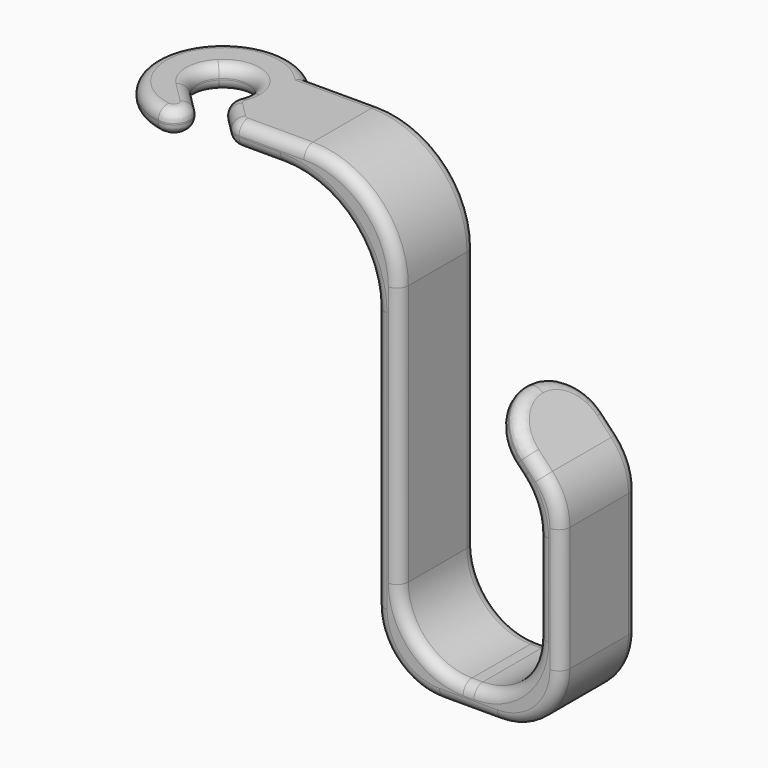
from build123d import *

# Parameters (mm, degrees)
F1_DEPTH = 15
F3_DEPTH = 7.4
F4_DEPTH = 25.4
F5_R     = 30
F6_R     = 20
F7_R     = 14.99999
F8_R     = 5.08
F9_R     = 3.5


# Not quite as in the source:
# - a fillet or chamfer is up to 0.001 mm smaller than in the source, because OpenCascade refuses the exact size


with BuildPart() as f1:
    # F0 (on Front) → F1 (new body, symmetric)
    with BuildSketch(Plane.XZ):
        Polygon((34.5196234971, 40.0508269668), (-48.0103765029, 40.0508269668), (-48.0103765029, 32.6508269668), (27.1196234971, 32.6508269668), (27.1196234971, -99.3991730332), (85.3275074601, -99.3991730332), (85.3275074601, -32.3411509969), (65.1577007475, -11.0187840781), (59.7818344831, -16.1040630192), (77.9275074601, -35.2866314352), (77.9275074601, -91.9991730332), (34.5196234971, -91.9991730332), align=None)
    extrude(amount=F1_DEPTH, both=True)

    # F2 (on face) → F3 (join)
    with BuildSketch(Plane.XY.offset(40.0508269668)):
        with BuildLine():
            Line((-17.993702875, 15), (-48.0103765029, 15))
            Line((-48.0103765029, 15), (-38.7238030188, 5.713423668))
            ThreePointArc((-38.7238030188, 5.713423668), (-29.918298397, 7.4649463856), (-24.9303811029, 0))
            ThreePointArc((-24.9303811029, 0), (-25.5454347172, -3.0920827058), (-27.2969591869, -5.713423668))
            Line((-27.2969591869, -5.713423668), (-18.0103857029, -15))
            Line((-18.0103857029, -15), (-17.993702875, -15))
            ThreePointArc((-17.993702875, -15), (-13.398782234, -8.1170077496), (-11.7853811029, 0))
            ThreePointArc((-11.7853811029, 0), (-13.398782234, 8.1170077496), (-17.993702875, 15))
        make_face()
        with BuildLine():
            Line((-38.7238030188, 5.713423668), (-48.0103765029, 15))
            Line((-48.0103765029, 15), (-48.0103765029, -15))
            Line((-48.0103765029, -15), (-38.7238030188, -5.713423668))
            ThreePointArc((-38.7238030188, -5.713423668), (-41.0903811029, 0), (-38.7238030188, 5.713423668))
        make_face()
        with BuildLine():
            Line((-48.0103765029, -15), (-48.0103765029, 15))
            Line((-48.0103765029, 15), (-17.993702875, 15))
            ThreePointArc((-17.993702875, 15), (-53.8308724589, 4.1240471255), (-24.8455044355, -19.5917179953))
            Line((-24.8455044355, -19.5917179953), (-29.437223839, -15))
            Line((-29.437223839, -15), (-48.0103765029, -15))
        make_face()
        Polygon((-38.7238030188, -5.713423668), (-48.0103765029, -15), (-29.437223839, -15), align=None)
    extrude(amount=-F3_DEPTH)

    # F2 (on face) → F4 (cut)
    with BuildSketch(Plane.XY.offset(40.0508269668)):
        with BuildLine():
            Line((-33.0103811029, 0), (-38.7238030188, -5.713423668))
            ThreePointArc((-38.7238030188, -5.713423668), (-33.0103811029, -8.08), (-27.2969591869, -5.713423668))
            Line((-27.2969591869, -5.713423668), (-33.0103811029, 0))
        make_face()
        with BuildLine():
            ThreePointArc((-24.9303811029, 0), (-29.918298397, 7.4649463856), (-38.7238030188, 5.713423668))
            Line((-38.7238030188, 5.713423668), (-33.0103811029, 0))
            Line((-33.0103811029, 0), (-27.2969591869, -5.713423668))
            ThreePointArc((-27.2969591869, -5.713423668), (-25.5454347172, -3.0920827058), (-24.9303811029, 0))
        make_face()
        with BuildLine():
            Line((-33.0103811029, 0), (-38.7238030188, 5.713423668))
            ThreePointArc((-38.7238030188, 5.713423668), (-41.0903811029, 0), (-38.7238030188, -5.713423668))
            Line((-38.7238030188, -5.713423668), (-33.0103811029, 0))
        make_face()
        with BuildLine():
            Line((-38.7238030188, -5.713423668), (-29.437223839, -15))
            Line((-29.437223839, -15), (-18.0103857029, -15))
            Line((-18.0103857029, -15), (-27.2969591869, -5.713423668))
            ThreePointArc((-27.2969591869, -5.713423668), (-33.0103811029, -8.08), (-38.7238030188, -5.713423668))
        make_face()
    extrude(amount=-F4_DEPTH, mode=Mode.SUBTRACT)

    # F5
    f5_edges = [f1.edges().sort_by_distance(p)[0] for p in [
        (34.519623, 0, 40.050827),
        (27.119623, 0, 32.650827),
    ]]
    fillet(f5_edges, radius=F5_R)

    # F6
    f6_edges = [f1.edges().sort_by_distance(p)[0] for p in [
        (27.119623, 0, -99.399173),
        (34.519623, 0, -91.999173),
        (85.327507, 0, -99.399173),
        (77.927507, 0, -91.999173),
        (77.927507, 0, -35.286631),
        (85.327507, 0, -32.341151),
    ]]
    fillet(f6_edges, radius=F6_R)

    # F7 (radius 15 in the source; OpenCascade refuses exactly that, so slightly less here)
    f7_edges = [f1.edges().sort_by_distance(p)[0] for p in [
        (62.469768, -15, -13.561424),
        (62.469768, 15, -13.561424),
    ]]
    fillet(f7_edges, radius=F7_R)

    # F8
    f8_edges = [f1.edges().sort_by_distance(p)[0] for p in [
        (-24.845504, -19.591718, 36.350827),
        (-27.296959, -5.713424, 36.350827),
        (-18.010386, -15, 36.350827),
    ]]
    fillet(f8_edges, radius=F8_R)

    # F9
    f9_edges = [f1.edges().sort_by_distance(p)[0] for p in [
        (-9.393278, -15, 32.650827),
        (-15.90618, -15, 36.350827),
        (18.332827, -15, 23.86403),
        (-5.693278, -15, 40.050827),
        (27.119623, -15, -38.374173),
        (25.732827, -15, 31.26403),
        (32.977488, -15, -93.541309),
        (34.519623, -15, -30.974173),
        (56.223565, -15, -99.399173),
        (40.377488, -15, -86.141309),
        (79.469643, -15, -93.541309),
        (56.223565, -15, -91.999173),
        (85.327507, -15, -59.850541),
        (72.069643, -15, -86.141309),
        (83.909587, -15, -32.905537),
        (77.927507, -15, -57.623281),
        (77.661284, -15, -24.236857),
        (76.509587, -15, -35.851017),
        (72.777759, -15, -24.458442),
        (71.273351, -15, -28.252237),
    ]]
    fillet(f9_edges, radius=F9_R)


solid = f1.part
